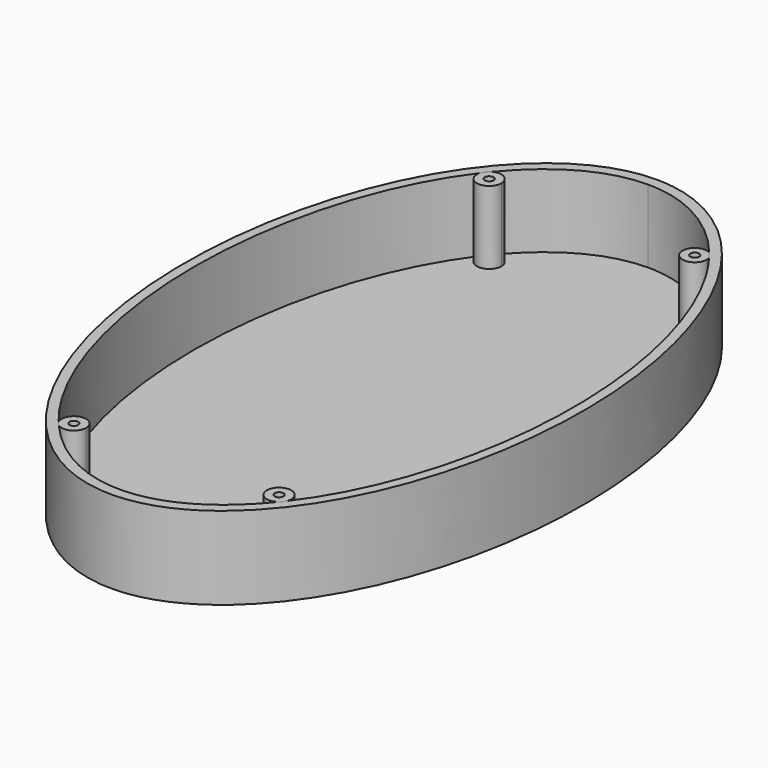
from build123d import *

# Parameters (mm, degrees)
F1_DEPTH  = 17
F3_DEPTH  = 15
F4_R      = 0.9
F5_DEPTH  = 15
F6_R      = 0.9
F7_DEPTH  = 15
F8_R      = 0.9
F9_DEPTH  = 15
F10_R     = 0.9
F11_DEPTH = 15
F13_R     = 0.9
F14_DEPTH = 17.0010001


with BuildPart() as f1:
    # F0 (on Top) → F1 (new body)
    with BuildSketch(Plane.XY):
        with BuildLine():
            add(Edge.make_bspline(
                [(-6.2171048485, 73.2565789297), (-77.2311879588, 73.2565789297), (-41.7241464036, -31.7434210703), (-6.2171048485, -136.7434210703), (29.2899367067, -31.7434210703), (64.7969782618, 73.2565789297), (-6.2171048485, 73.2565789297)],
                knots=[0, 0, 0, 2.0943951024, 2.0943951024, 4.1887902048, 4.1887902048, 6.2831853072, 6.2831853072, 6.2831853072], degree=2, weights=[1, 0.5, 1, 0.5, 1, 0.5, 1]))
        make_face()
    extrude(amount=F1_DEPTH)

    # F2 (on face) → F3 (cut)
    with BuildSketch(Plane.XY.offset(17)):
        with BuildLine():
            add(Edge.make_bspline(
                [(-6.2171048485, 71.0526332259), (-73.7670863437, 71.0526332259), (-39.9920955961, -30.6414482184), (-6.2171048485, -132.3355296627), (27.5578858991, -30.6414482184), (61.3328766467, 71.0526332259), (-6.2171048485, 71.0526332259)],
                knots=[0, 0, 0, 2.0943951024, 2.0943951024, 4.1887902048, 4.1887902048, 6.2831853072, 6.2831853072, 6.2831853072], degree=2, weights=[1, 0.5, 1, 0.5, 1, 0.5, 1]))
        make_face()
    extrude(amount=-F3_DEPTH, mode=Mode.SUBTRACT)

    # F4 (on face) → F5 (join)
    with BuildSketch(Plane.XY.offset(2)):
        with BuildLine():
            ThreePointArc((-29.7756858862, 57.2855702673), (-27.6492449133, 54.2060390081), (-24.8481921157, 56.6878462554))
            ThreePointArc((-24.8481921157, 56.6878462554), (-26.0432758657, 58.8202612198), (-28.48594698, 58.9139446065))
            add(Edge.make_bspline(
                [(-28.48594698, 58.9139446065), (-29.1403899926, 58.1226714215), (-29.7756858862, 57.2855702673)],
                knots=[0.6420928407, 0.6420928407, 0.6420928407, 0.6808401148, 0.6808401148, 0.6808401148], degree=2, weights=[0.7874125542, 0.783834135, 0.7805979828]))
        make_face()
        with Locations((-27.3481921157, 56.6878462554)):
            Circle(F4_R, mode=Mode.SUBTRACT)
        with BuildLine():
            add(Edge.make_bspline(
                [(-28.48594698, 58.9139446065), (-29.1403899926, 58.1226714215), (-29.7756858862, 57.2855702673)],
                knots=[0.6420928407, 0.6420928407, 0.6420928407, 0.6808401148, 0.6808401148, 0.6808401148], degree=2, weights=[0.7874125542, 0.783834135, 0.7805979828]))
            ThreePointArc((-28.48594698, 58.9139446065), (-29.3079498058, 58.2400542943), (-29.7756858862, 57.2855702673))
        make_face()
    extrude(amount=F5_DEPTH)

    # F6 (on face) → F7 (join)
    with BuildSketch(Plane.XY.offset(2)):
        with BuildLine():
            ThreePointArc((16.1916939477, 58.7439345546), (12.7793422864, 55.3266057789), (17.4437982507, 56.577657488))
            ThreePointArc((17.4437982507, 56.577657488), (17.4180855063, 56.9352921855), (17.3414761892, 57.2855702673))
            add(Edge.make_bspline(
                [(17.3414761892, 57.2855702673), (16.7742405528, 58.0329914466), (16.1916939477, 58.7439345546)],
                knots=[5.6023451924, 5.6023451924, 5.6023451924, 5.6369260508, 5.6369260508, 5.6369260508], degree=2, weights=[0.7805979828, 0.7834861581, 0.7866469513]))
        make_face()
        with Locations((14.9437982507, 56.577657488)):
            Circle(F6_R, mode=Mode.SUBTRACT)
    extrude(amount=F7_DEPTH)

    # F8 (on face) → F9 (join)
    with BuildSketch(Plane.XY.offset(2)):
        with BuildLine():
            ThreePointArc((-27.8172974331, -53.191482885), (-25.1847662143, -53.4621797963), (-23.7840667271, -51.2168427654))
            ThreePointArc((-23.7840667271, -51.2168427654), (-26.8945171213, -48.792518052), (-28.48594698, -52.4007867471))
            add(Edge.make_bspline(
                [(-28.48594698, -52.4007867471), (-28.1539802485, -52.8021606908), (-27.8172974331, -53.191482885)],
                knots=[2.5728398269, 2.5728398269, 2.5728398269, 2.5934282254, 2.5934282254, 2.5934282254], degree=2, weights=[0.8237445465, 0.8210750527, 0.8185021925]))
        make_face()
        with Locations((-26.2840667271, -51.2168427654)):
            Circle(F8_R, mode=Mode.SUBTRACT)
    extrude(amount=F9_DEPTH)

    # F10 (on face) → F11 (join)
    with BuildSketch(Plane.XY.offset(2)):
        with BuildLine():
            ThreePointArc((17.2071260982, -50.948647347), (17.3423414514, -50.4905518475), (17.3879683871, -50.0151016807))
            ThreePointArc((17.3879683871, -50.0151016807), (12.6660564501, -48.8691927208), (16.3374825114, -52.0519887181))
            add(Edge.make_bspline(
                [(16.3374825114, -52.0519887181), (16.7766850943, -51.5107523345), (17.2071260982, -50.948647347)],
                knots=[3.7192756497, 3.7192756497, 3.7192756497, 3.746975358, 3.746975358, 3.746975358], degree=2, weights=[0.8260785, 0.8297264389, 0.8335492953]))
        make_face()
        with Locations((14.8879683871, -50.0151016807)):
            Circle(F10_R, mode=Mode.SUBTRACT)
        with BuildLine():
            add(Edge.make_bspline(
                [(16.3374825114, -52.0519887181), (16.7766850943, -51.5107523345), (17.2071260982, -50.948647347)],
                knots=[3.7192756497, 3.7192756497, 3.7192756497, 3.746975358, 3.746975358, 3.746975358], degree=2, weights=[0.8260785, 0.8297264389, 0.8335492953]))
            ThreePointArc((16.3374825114, -52.0519887181), (16.8513996683, -51.5626602753), (17.2071260982, -50.948647347))
        make_face()
    extrude(amount=F11_DEPTH)

    # F13 (on face) → F14 (cut, through all)
    with BuildSketch(Plane.XY.offset(17)):
        with Locations((-27.3481921157, 56.6878462554)):
            Circle(F13_R)
        with Locations((14.9437982507, 56.577657488)):
            Circle(F13_R)
        with Locations((-26.2840667271, -51.2168427654)):
            Circle(F13_R)
        with Locations((14.8879683871, -50.0151016807)):
            Circle(F13_R)
    extrude(amount=-F14_DEPTH, mode=Mode.SUBTRACT)


solid = f1.part
